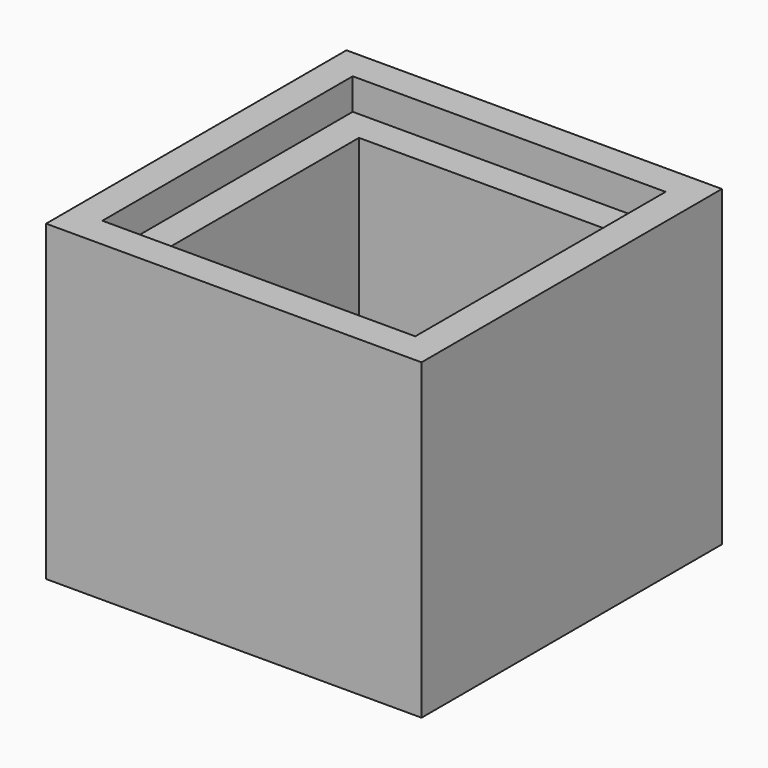
from build123d import *

# Parameters (mm, degrees)
F0_W     = 60
F0_H     = 60
F1_DEPTH = 50
F2_W     = 40
F2_H     = 40
F3_DEPTH = 40
F4_W     = 50
F4_H     = 50
F5_DEPTH = 5


# Not quite as in the source:
# - a feature names something its author has since deleted; it is built from what else it names


with BuildPart() as f1:
    # F0 (on Top) → F1 (new body)
    with BuildSketch(Plane.XY):
        with Locations((30, 30)):
            Rectangle(F0_W, F0_H)
    extrude(amount=-F1_DEPTH)

    # F2 (on Top) → F3 (cut)
    with BuildSketch(Plane.XY):
        with Locations((30, 30)):
            Rectangle(F2_W, F2_H)
    extrude(amount=-F3_DEPTH, mode=Mode.SUBTRACT)

    # F4 (on Top) → F5 (cut)
    with BuildSketch(Plane.XY):
        with Locations((30, 30)):
            Rectangle(F4_W, F4_H)
    extrude(amount=-F5_DEPTH, mode=Mode.SUBTRACT)


solid = f1.part
